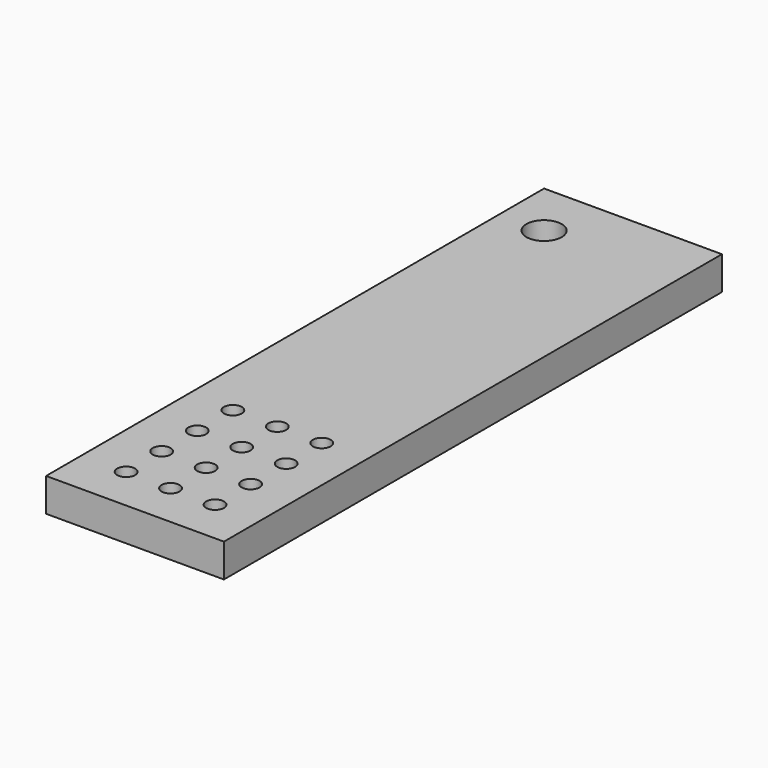
from build123d import *

# Parameters (mm, degrees)
F0_W     = 50.8
F0_H     = 177.8
F1_DEPTH = 9.525
F2_D     = 5.1054
F3_D     = 10.0838


# Not quite as in the source:
# - a length typed as a fraction of an inch, garbled in the dataset ("3 / 203.2 mm" for 3/8 in), is restored


with BuildPart() as f1:
    # F0 (on Top) → F1 (new body)
    with BuildSketch(Plane.XY):
        with Locations((-25.4, 88.9)):
            Rectangle(F0_W, F0_H)
    extrude(amount=-F1_DEPTH)

    # F2 (through all)
    with Locations(Plane.XY):
        with Locations((-12.7, 12.7), (-25.4, 12.7), (-38.1, 12.7), (-38.1, 25.4), (-25.4, 25.4), (-12.7, 25.4), (-12.7, 38.1), (-25.4, 38.1), (-38.1, 38.1), (-38.1, 50.8), (-25.4, 50.8), (-12.7, 50.8)):
            Hole(F2_D / 2)

    # F3 (through all)
    with Locations(Plane.XY):
        with Locations((-38.1, 161.925)):
            Hole(F3_D / 2)


solid = f1.part
